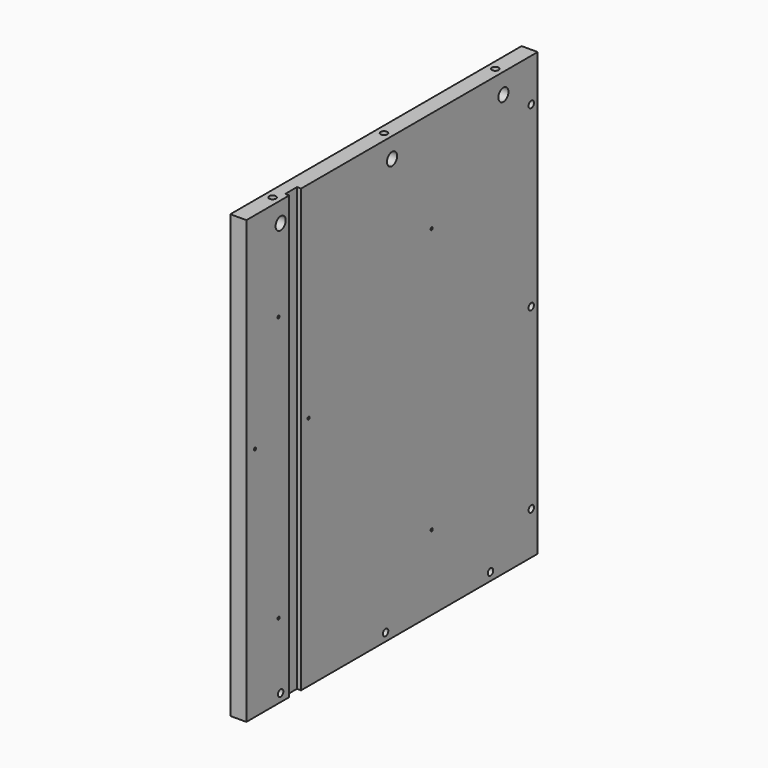
from build123d import *

# Parameters (mm, degrees)
F0_W      = 431.8
F0_H      = 523.875
F1_DEPTH  = 19.05
F3_D      = 8.001
F3_DEPTH  = 14.224
F3_TIP    = 2.4037429064
F4_D      = 15.0114
F4_DEPTH  = 14.224
F4_TIP    = 4.5098795482
F6_D      = 8.001
F6_DEPTH  = 25.4
F6_TIP    = 2.4037429064
F8_D      = 3.175
F8_DEPTH  = 14.224
F8_TIP    = 0.9538662327
F9_W      = 17.526
F9_H      = 523.875
F10_DEPTH = 4.826


with BuildPart() as f1:
    # F0 (on Right) → F1 (new body)
    with BuildSketch(Plane.YZ):
        Rectangle(F0_W, F0_H)
    extrude(amount=F1_DEPTH)

    # F3
    with Locations(Plane.YZ.offset(19.05)):
        with Locations((206.375, 211.1375), (206.375, -211.1375), (146.05, -252.4125), (-9.525, -252.4125), (-165.1, -252.4125), (206.375, 0)):
            Hole(F3_D / 2, depth=F3_DEPTH)
            with Locations((0, 0, -(F3_DEPTH + F3_TIP / 2))):  # 118° drill point
                Cone(0, F3_D / 2, F3_TIP, mode=Mode.SUBTRACT)

    # F4
    with Locations(Plane.YZ.offset(19.05)):
        with Locations((-165.1, 238.0615), (0, 238.0615), (165.1, 238.0615)):
            Hole(F4_D / 2, depth=F4_DEPTH)
            with Locations((0, 0, -(F4_DEPTH + F4_TIP / 2))):  # 118° drill point
                Cone(0, F4_D / 2, F4_TIP, mode=Mode.SUBTRACT)

    # F6
    with Locations(Plane.XY.offset(261.9375)):
        with Locations((9.525, 165.1), (9.525, 0), (9.525, -165.1)):
            Hole(F6_D / 2, depth=F6_DEPTH)
            with Locations((0, 0, -(F6_DEPTH + F6_TIP / 2))):  # 118° drill point
                Cone(0, F6_D / 2, F6_TIP, mode=Mode.SUBTRACT)

    # F8
    with Locations(Plane.YZ.offset(19.05)):
        with Locations((-168.275, 141.4145), (58.7375, 141.4145), (-203.2, 17.7165), (-123.825, 17.7165), (-168.275, -173.0375), (58.7375, -173.0375)):
            Hole(F8_D / 2, depth=F8_DEPTH)
            with Locations((0, 0, -(F8_DEPTH + F8_TIP / 2))):  # 118° drill point
                Cone(0, F8_D / 2, F8_TIP, mode=Mode.SUBTRACT)

    # F9 (on face) → F10 (cut)
    with BuildSketch(Plane.YZ.offset(19.05)):
        with Locations((-143.637, 0)):
            Rectangle(F9_W, F9_H)
    extrude(amount=-F10_DEPTH, mode=Mode.SUBTRACT)


solid = f1.part
